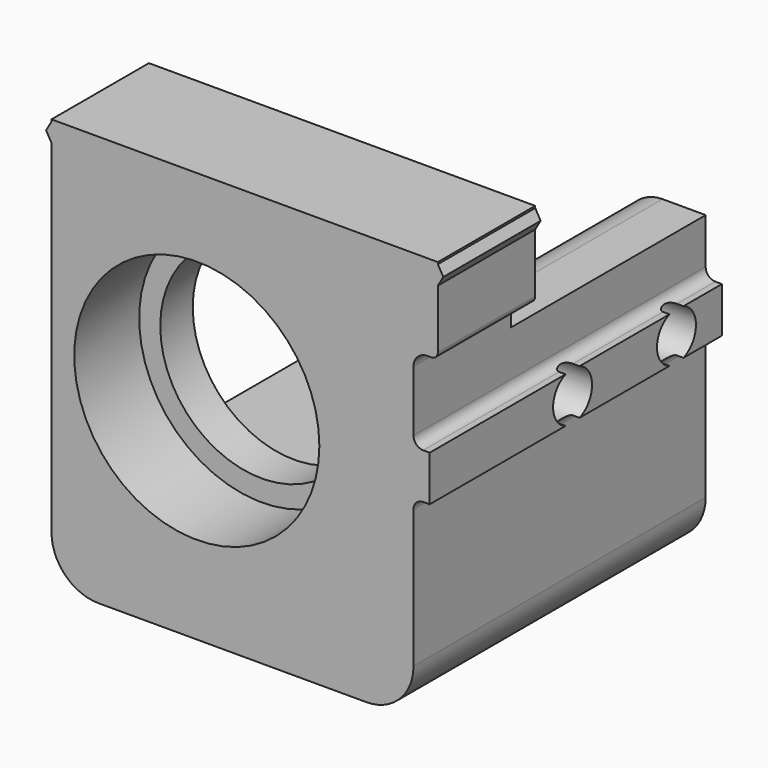
from build123d import *

# Parameters (mm, degrees)
F1_DEPTH  = 55
F3_DEPTH  = 30
F4_R      = 3
F5_DEPTH  = 25
F6_R      = 12.5
F7_DEPTH  = 55.0010001
F8_R      = 15.1
F9_DEPTH  = 20
F10_R     = 6.5
F11_DEPTH = 17
F12_R     = 10
F13_W     = 62.573639676
F13_H     = 57.5273763388
F14_DEPTH = 10


# Not quite as in the source:
# - a feature names something its author has since deleted; it is built from what else it names


with BuildPart() as f1:
    # F0 (on Front) → F1 (new body)
    with BuildSketch(Plane.XZ):
        with BuildLine():
            Line((-23.6999987811, 23.7999986857), (-23.6999987811, 23.5588453133))
            Line((-23.6999987811, 23.5588453133), (-24.3690585991, 22.3999992996))
            Line((-24.3690585991, 22.3999992996), (-23.6999987811, 21.241153286))
            Line((-23.6999987811, 21.241153286), (-23.6999987811, -21.0000007004))
            ThreePointArc((-23.6999987811, -21.0000007004), (-22.0012182918, -25.1012195971), (-17.899999395, -26.8000000864))
            Line((-17.899999395, -26.8000000864), (15.100000605, -26.8000000864))
            ThreePointArc((15.100000605, -26.8000000864), (19.2012195018, -25.1012195971), (20.8999999911, -21.0000007004))
            Line((20.8999999911, -21.0000007004), (20.8999999911, -4.0000007004))
            ThreePointArc((20.8999999911, -4.0000007004), (21.2514720335, -3.1514721288), (22.100000605, -2.8000000864))
            Line((22.100000605, -2.8000000864), (22.8999999911, -2.8000000864))
            Line((22.8999999911, -2.8000000864), (22.8999999911, 2.7999986857))
            Line((22.8999999911, 2.7999986857), (22.100000605, 2.7999986857))
            ThreePointArc((22.100000605, 2.7999986857), (21.2514720335, 3.1514707281), (20.8999999911, 3.9999992996))
            Line((20.8999999911, 3.9999992996), (20.8999999911, 11.4999992996))
            ThreePointArc((20.8999999911, 11.4999992996), (21.3979186429, 12.7020812618), (22.600000605, 13.1999999136))
            Line((22.600000605, 13.1999999136), (23.100000605, 13.1999999136))
            ThreePointArc((23.100000605, 13.1999999136), (23.6656855958, 13.4343143088), (23.8999999911, 13.9999992996))
            Line((23.8999999911, 13.9999992996), (23.8999999911, 21.241153286))
            Line((23.8999999911, 21.241153286), (24.5690598091, 22.3999992996))
            Line((24.5690598091, 22.3999992996), (23.8999999911, 23.5588453133))
            Line((23.8999999911, 23.5588453133), (23.8999999911, 23.7999986857))
            Line((23.8999999911, 23.7999986857), (-23.6999987811, 23.7999986857))
        make_face()
    extrude(amount=F1_DEPTH)

    # F2 (on face) → F3 (cut)
    with BuildSketch(Plane(origin=(0, 0, 0), x_dir=(-1, 0, 0), z_dir=(0, 1, 0))):
        with BuildLine():
            Line((-9.7267732358, -17.8000000864), (27.0197465134, -17.8000000864))
            Line((27.0197465134, -17.8000000864), (27.0197465134, 29.101931586))
            Line((27.0197465134, 29.101931586), (-25.6962114531, 29.101931586))
            Line((-25.6962114531, 29.101931586), (-25.6962114531, 9.6292318066))
            Line((-25.6962114531, 9.6292318066), (-15.5874993246, 9.6292318066))
            ThreePointArc((-15.5874993246, 9.6292318066), (-12.272936759, 8.2562950386), (-10.8999999911, 4.9417324731))
            Line((-10.8999999911, 4.9417324731), (-10.8999999911, -12.1750008862))
            Line((-10.8999999911, -12.1750008862), (-10.8999999911, -17.8000000864))
            Line((-10.8999999911, -17.8000000864), (-9.7267732358, -17.8000000864))
        make_face()
    extrude(amount=-F3_DEPTH, mode=Mode.SUBTRACT)

    # F4 (on face) → F5 (cut)
    with BuildSketch(Plane.YZ.offset(22.8999999911)):
        with Locations((-7, -1.3143e-06)):
            Circle(F4_R)
        with Locations((-23, -1.3143e-06)):
            Circle(F4_R)
    extrude(amount=-F5_DEPTH, mode=Mode.SUBTRACT)

    # F6 (on face) → F7 (cut, through all)
    with BuildSketch(Plane(origin=(0, 0, 0), x_dir=(-1, 0, 0), z_dir=(0, 1, 0))):
        with Locations((5.7999987811, -0.9000000864)):
            Circle(F6_R)
    extrude(amount=-F7_DEPTH, mode=Mode.SUBTRACT)

    # F8 (on face) → F9 (cut)
    with BuildSketch(Plane.XZ.offset(55)):
        with Locations((-5.7999987811, -0.9000000864)):
            Circle(F8_R)
    extrude(amount=-F9_DEPTH, mode=Mode.SUBTRACT)

    # F10 (on Right) → F11 (cut)
    with BuildSketch(Plane.YZ):
        with Locations((-23, 0)):
            Circle(F10_R)
        with Locations((-7, 0)):
            Circle(F10_R)
    extrude(amount=F11_DEPTH, mode=Mode.SUBTRACT)

    # F12
    f12_edges = [f1.edges().sort_by_distance(p)[0] for p in [
        (10.9, -15, -17.8),
    ]]
    fillet(f12_edges, radius=F12_R)

    # F13 (on face) → F14 (cut)
    with BuildSketch(Plane.XZ.offset(55)):
        with Locations((1.9923495129, 0.0138776377)):
            Rectangle(F13_W, F13_H)
    extrude(amount=-F14_DEPTH, mode=Mode.SUBTRACT)


solid = f1.part
